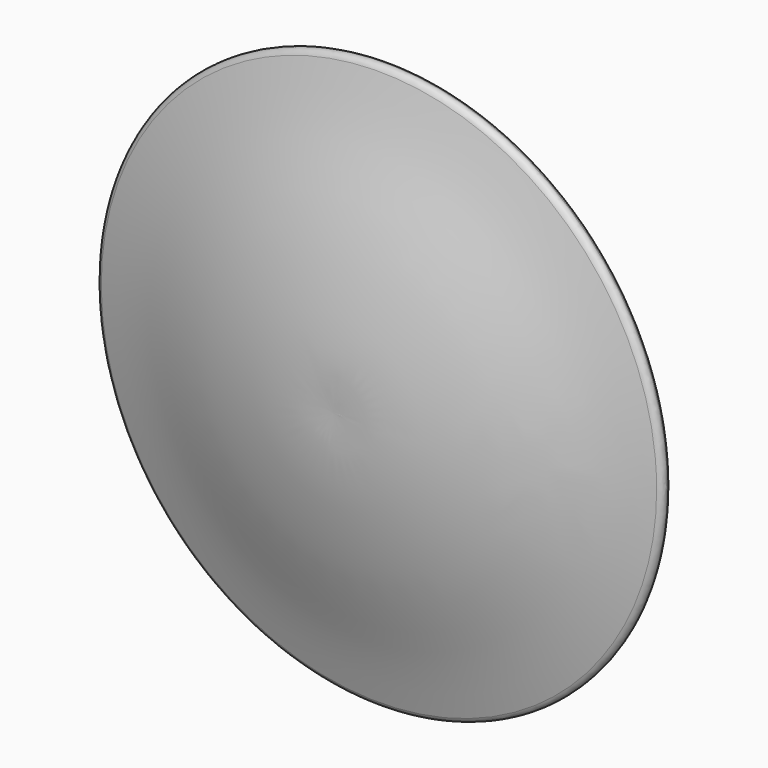
from build123d import *

# Parameters (mm, degrees)
F4_R = 1.524


# Not quite as in the source:
# - a feature of the source that left no trace in its solid (it failed there, or was rolled back) is left out
# - the dataset's text gives a spline's control points without its knots; the knots are read off the source's solid


with BuildPart() as f1:
    # F0 (on Top) → F1 (revolve)
    with BuildSketch(Plane.XY):
        with BuildLine():
            Line((0, 3.175), (0, 0))
            add(Edge.make_bspline(
                [(0, 0), (0.9391765667, 0), (2.8722299911, -0.0522262833), (6.170117236, -0.1441224404), (9.3929267103, -0.0927233382), (12.3370917537, 0.1121304597), (15.4679032393, 0.4237260784), (19.6887306562, 0.9960590173), (25.0468368551, 1.9343747406), (29.5844448409, 2.8927642781), (33.1525403626, 3.7458266346), (36.6468404962, 4.6519123387), (40.7910006378, 5.8602443837), (45.4421011997, 7.3523485387), (49.8066693073, 8.8119965269), (53.2361141861, 9.9414244239), (55.8678215732, 10.7548261199), (58.4617485931, 11.5143988036), (61.6444560074, 12.380341327), (65.4120841236, 13.3316057251), (67.916879148, 13.9383668447), (69.1740895707, 14.2426631846)],
                knots=[0, 0, 0, 0, 0.0625, 0.125, 0.1875, 0.21875, 0.25, 0.3125, 0.375, 0.4375, 0.46875, 0.5, 0.5625, 0.625, 0.6875, 0.75, 0.78125, 0.8125, 0.875, 0.9375, 1, 1, 1, 1], degree=3))
            Line((69.1740895707, 14.2426631846), (68.4271768355, 17.3285579277))
            add(Edge.make_bspline(
                [(0, 3.175), (3.1284372612, 3.175), (10.9563662678, 2.5008036316), (34.8837140717, 6.7254308845), (53.5336074809, 13.7166970204), (63.7395760718, 16.1939668287), (68.4271768355, 17.3285579277)],
                knots=[0, 0, 0, 0, 0.1961119482, 0.4928846131, 0.767030546, 1, 1, 1, 1], degree=3))
        make_face()
    revolve(axis=Axis((0, 1.5875, 0), (0, 1, 0)))

    # F4
    f4_edges = [f1.edges().sort_by_distance(p)[0] for p in [
        (-68.427177, 17.328558, 0),
        (-69.17409, 14.242663, 0),
    ]]
    fillet(f4_edges, radius=F4_R)


solid = f1.part
